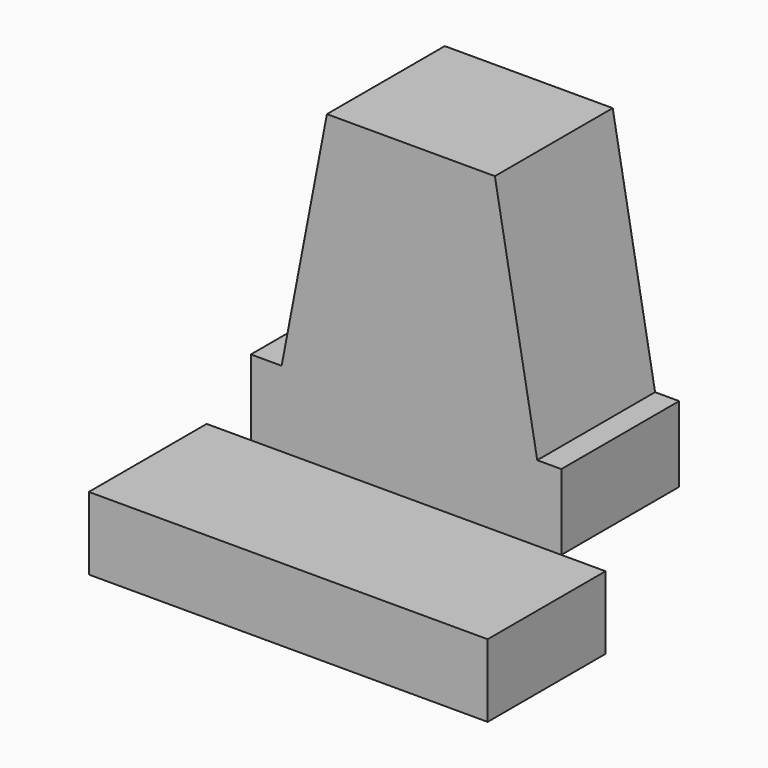
from build123d import *

# Parameters (mm, degrees)
F1_DEPTH = 50.8
F3_DEPTH = 25.4
F5_DEPTH = 25.4


with BuildPart() as f1:
    # F0 (on Front) → F1 (new body)
    with BuildSketch(Plane.XZ):
        Polygon((-120.0167089701, 26.0464213789), (-130.6295543909, 26.0464213789), (-130.6295543909, 0), (-23.5658083111, 0), (-23.5658083111, 26.0464213789), (-31.8762026727, 26.0464213789), align=None)
        Polygon((-104.4032499194, 107.5314208865), (-120.0167089701, 26.0464213789), (-31.8762026727, 26.0464213789), (-46.4823432267, 107.5314208865), align=None)
    extrude(amount=F1_DEPTH)


with BuildPart() as f3:
    # F2 (on face) → F3 (new body)
    with BuildSketch(Plane.XZ.offset(50.8)):
        Polygon((-23.5658083111, 0), (-130.6295543909, 0), (-145.8695543909, 0), (-145.8695543909, -25.1038316637), (-8.3258083111, -25.1038316637), (-8.3258083111, 0), align=None)
    extrude(amount=F3_DEPTH)

    # F5 (add): a face of the model
    f5_faces = [f3.faces().sort_by_distance(p)[0] for p in [
        (-77.097681351, -76.2, -12.5519158319),
    ]]
    extrude(f5_faces, amount=F5_DEPTH)


solid = Compound([f1.part, f3.part])
